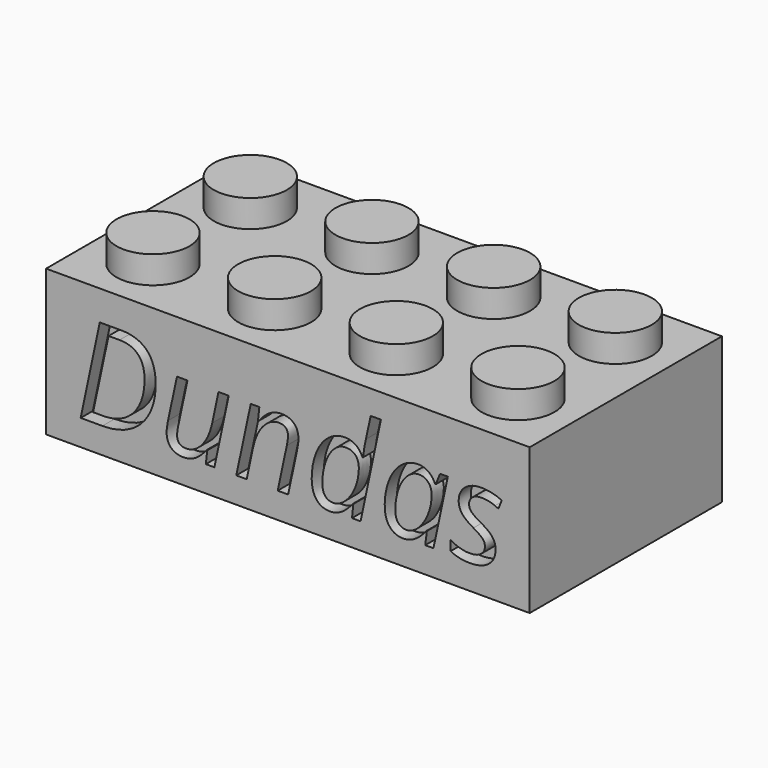
from build123d import *

# Parameters (mm, degrees)
F0_W          = 31.8
F0_H          = 15.8
F1_DEPTH      = 9.6
F2_W          = 29.4
F2_H          = 13.4
F3_DEPTH      = 8.4
F4_R          = 2.4
F5_DEPTH      = 1.8
F6_R          = 1.3
F7_DEPTH      = 1.2
F8_TEXT_SIZE  = 8.3174913824
F9_DEPTH      = 1
F10_TEXT_SIZE = 7.2084920248
F11_DEPTH     = 1
F12_W         = 0.6
F12_H         = 0.3
F13_DEPTH     = 8.4
F14_W         = 0.3
F14_H         = 0.6
F15_DEPTH     = 8.4
F16_W         = 0.6
F16_H         = 3.4669781491
F16_H_2       = 3.5
F17_DEPTH     = 6.4
F18_R         = 3.255
F18_R_2       = 2.4
F19_DEPTH     = 8.4


# Not quite as in the source:
# - Text() gives the source's letters only with a copy of the font that has no kerning and outlines rounded to 1/6400 em; it was checked with that copy


with BuildPart() as f1:
    # F0 (on Top) → F1 (new body)
    with BuildSketch(Plane.XY):
        Rectangle(F0_W, F0_H)
    extrude(amount=F1_DEPTH)

    # F2 (on Top) → F3 (cut)
    with BuildSketch(Plane.XY):
        Rectangle(F2_W, F2_H)
    extrude(amount=F3_DEPTH, mode=Mode.SUBTRACT)

    # F4 (on face) → F5 (join)
    with BuildSketch(Plane.XY.offset(9.6)):
        with Locations((-11.95, 3.95)):
            Circle(F4_R)
        with Locations((-11.95, -4.05)):
            Circle(F4_R)
        with Locations((-3.95, 3.95)):
            Circle(F4_R)
        with Locations((-3.95, -4.05)):
            Circle(F4_R)
        with Locations((4.05, 3.95)):
            Circle(F4_R)
        with Locations((4.05, -4.05)):
            Circle(F4_R)
        with Locations((12.05, 3.95)):
            Circle(F4_R)
        with Locations((12.05, -4.05)):
            Circle(F4_R)
    extrude(amount=F5_DEPTH)

    # F6 (on face) → F7 (cut)
    with BuildSketch(Plane(origin=(0, 0, 8.4), x_dir=(1, 0, 0), z_dir=(0, 0, -1))):
        with Locations((-11.95, 3.95)):
            Circle(F6_R)
        with Locations((-11.95, -4.05)):
            Circle(F6_R)
        with Locations((-3.95, 3.95)):
            Circle(F6_R)
        with Locations((-3.95, -4.05)):
            Circle(F6_R)
        with Locations((4.05, 3.95)):
            Circle(F6_R)
        with Locations((4.05, -4.05)):
            Circle(F6_R)
        with Locations((12.05, 3.95)):
            Circle(F6_R)
        with Locations((12.05, -4.05)):
            Circle(F6_R)
    extrude(amount=-F7_DEPTH, mode=Mode.SUBTRACT)

    # F8 (on face) → F9 (cut)
    with BuildSketch(Plane.XZ.offset(7.9)):
        with Locations((-13.9733841643, 1.6967681004)):
            Text('Dundas', F8_TEXT_SIZE, font='Open Sans', font_style=FontStyle.ITALIC, text_align=(TextAlign.LEFT, TextAlign.BOTTOM))
    extrude(amount=-F9_DEPTH, mode=Mode.SUBTRACT)

    # F10 (on face) → F11 (cut)
    with BuildSketch(Plane(origin=(0, 7.9, 0), x_dir=(-1, 0, 0), z_dir=(0, 1, 0))):
        with Locations((-7.585552521, 2.0960078109)):
            Text('2018', F10_TEXT_SIZE, font='Open Sans', font_style=FontStyle.ITALIC, text_align=(TextAlign.LEFT, TextAlign.BOTTOM))
    extrude(amount=-F11_DEPTH, mode=Mode.SUBTRACT)

    # F12 (on face) → F13 (join, through all)
    with BuildSketch(Plane(origin=(0, 0, 0), x_dir=(1, 0, 0), z_dir=(0, 0, -1))):
        with Locations((-11.95, 6.55)):
            Rectangle(F12_W, F12_H)
        with Locations((-11.95, -6.55)):
            Rectangle(F12_W, F12_H)
        with Locations((-3.95, 6.55)):
            Rectangle(F12_W, F12_H)
        with Locations((-3.95, -6.55)):
            Rectangle(F12_W, F12_H)
        with Locations((4.05, 6.55)):
            Rectangle(F12_W, F12_H)
        with Locations((4.05, -6.55)):
            Rectangle(F12_W, F12_H)
        with Locations((12.05, 6.55)):
            Rectangle(F12_W, F12_H)
        with Locations((12.05, -6.55)):
            Rectangle(F12_W, F12_H)
    extrude(amount=-F13_DEPTH)

    # F14 (on face) → F15 (join)
    with BuildSketch(Plane(origin=(0, 0, 8.4), x_dir=(1, 0, 0), z_dir=(0, 0, -1))):
        with Locations((-14.55, -3.95)):
            Rectangle(F14_W, F14_H)
        with Locations((-14.55, 4.05)):
            Rectangle(F14_W, F14_H)
        with Locations((14.55, -3.95)):
            Rectangle(F14_W, F14_H)
        with Locations((14.55, 4.05)):
            Rectangle(F14_W, F14_H)
    extrude(amount=F15_DEPTH)

    # F16 (on face) → F17 (join)
    with BuildSketch(Plane(origin=(0, 0, 8.4), x_dir=(1, 0, 0), z_dir=(0, 0, -1))):
        with Locations((0, -4.9665109254)):
            Rectangle(F16_W, F16_H)
        with Locations((0, 4.95)):
            Rectangle(F16_W, F16_H_2)
    extrude(amount=F17_DEPTH)

    # F18 (on face) → F19 (join, through all)
    with BuildSketch(Plane(origin=(0, 0, 8.4), x_dir=(1, 0, 0), z_dir=(0, 0, -1))):
        with Locations((-7.95, -0.05)):
            Circle(F18_R)
        with Locations((-7.95, -0.05)):
            Circle(F18_R_2, mode=Mode.SUBTRACT)
        with Locations((0.05, -0.05)):
            Circle(F18_R)
        with Locations((0.05, -0.05)):
            Circle(F18_R_2, mode=Mode.SUBTRACT)
        with Locations((8.05, -0.05)):
            Circle(F18_R)
        with Locations((8.05, -0.05)):
            Circle(F18_R_2, mode=Mode.SUBTRACT)
    extrude(amount=F19_DEPTH)


solid = f1.part
